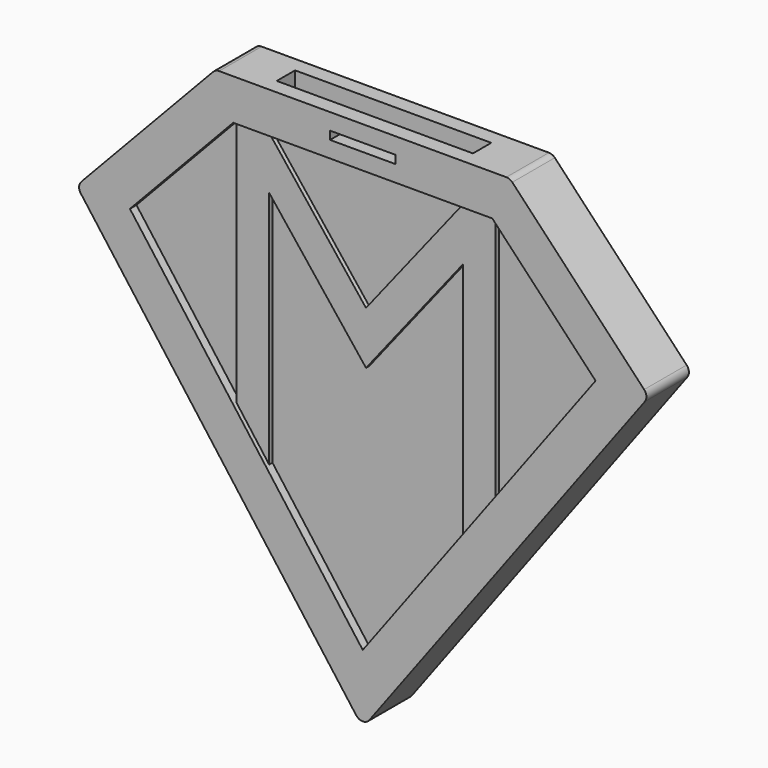
from build123d import *

# Parameters (mm, degrees)
F1_DEPTH  = 3.25
F3_DEPTH  = 0.5
F5_DEPTH  = 0.5
F7_DEPTH  = 0.5
F9_DEPTH  = 0.5
F10_W     = 24
F10_H     = 2.8
F11_DEPTH = 20
F13_DEPTH = 1.4
F14_W     = 8
F14_H     = 1
F15_DEPTH = 25
F16_R     = 1


# Not quite as in the source:
# - ends of sketch curves that miss each other by under 0.0002 mm in the source are joined


with BuildPart() as f1:
    # F0 (on Front) → F1 (new body, symmetric)
    with BuildSketch(Plane.XZ):
        Polygon((18, 18), (0, 18), (-18, 18), (-35, 0), (0, -47), (35, 0), align=None)
    extrude(amount=F1_DEPTH, both=True)

    # F2 (on face) → F3 (cut)
    with BuildSketch(Plane.XZ.offset(3.25)):
        Polygon((15.8447675538, 13), (-15.8447675538, 13), (-28.4822773709, -0.3808927475), (1.162e-07, -38.628522516), (28.4822775009, -0.3808928851), align=None)
    extrude(amount=-F3_DEPTH, mode=Mode.SUBTRACT)

    # F4 (on face) → F5 (cut)
    with BuildSketch(Plane(origin=(0, 3.25, 0), x_dir=(-1, 0, 0), z_dir=(0, 1, 0))):
        Polygon((28.482277527, -0.3808925379), (15.8447676545, 13.0000002682), (-15.8447670441, 13.0000002682), (-28.4822772579, -0.3808928993), (0, -38.6285223599), align=None)
    extrude(amount=-F5_DEPTH, mode=Mode.SUBTRACT)

    # F6 (on face) → F7 (cut)
    with BuildSketch(Plane.XZ.offset(2.75)):
        Polygon((-15.8447675538, -17.3512630734), (-15.8447675538, 13), (-28.4822773709, -0.3808927475), align=None)
        Polygon((28.4822775009, -0.3808928851), (15.8447675538, 13), (15.8447675538, -17.3512633855), align=None)
        Polygon((0, -8.4544227059), (-11.8447675538, 6.5455772941), (-11.8447675538, -22.7226916448), (1.162e-07, -38.628522516), (11.8447675538, -22.7226919569), (11.8447675538, 6.5455772941), align=None)
        Polygon((11.8447675538, 13), (-11.8447675538, 13), (0, -2), align=None)
    extrude(amount=-F7_DEPTH, mode=Mode.SUBTRACT)

    # F8 (on face) → F9 (cut)
    with BuildSketch(Plane(origin=(0, 2.75, 0), x_dir=(-1, 0, 0), z_dir=(0, 1, 0))):
        Polygon((-15.8447675538, -17.3512633855), (-15.8447675538, 13), (-28.4822772579, -0.3808928993), align=None)
        Polygon((0, -8.4544227059), (-11.8447675538, 6.5455772941), (-11.8447675538, -22.7226919569), (0, -38.6285223599), (11.8447675538, -22.7226916448), (11.8447675538, 6.5455772941), align=None)
        Polygon((-11.8447675538, 13), (0, -2), (11.8447675538, 13), align=None)
        Polygon((28.482277527, -0.3808925379), (15.8447676545, 13.0000002682), (15.8447675538, -17.3512630734), align=None)
    extrude(amount=-F9_DEPTH, mode=Mode.SUBTRACT)

    # F10 (on face) → F11 (cut)
    with BuildSketch(Plane.XY.offset(18)):
        Rectangle(F10_W, F10_H)
    extrude(amount=-F11_DEPTH, mode=Mode.SUBTRACT)

    # F12 (on Front) → F13 (cut, symmetric)
    with BuildSketch(Plane.XZ):
        with BuildLine():
            Line((12, -2), (-12, -2))
            ThreePointArc((-12, -2), (0, -14), (12, -2))
        make_face()
    extrude(amount=F13_DEPTH, both=True, mode=Mode.SUBTRACT)

    # F14 (on face) → F15 (cut)
    with BuildSketch(Plane.XZ.offset(3.25)):
        with Locations((0, 15.5)):
            Rectangle(F14_W, F14_H)
    extrude(amount=-F15_DEPTH, mode=Mode.SUBTRACT)

    # F16
    f16_edges = [f1.edges().sort_by_distance(p)[0] for p in [
        (0, 0, -47),
        (35, 0, 0),
        (-35, 0, 0),
        (-18, 0, 18),
        (18, 0, 18),
    ]]
    fillet(f16_edges, radius=F16_R)


solid = f1.part
